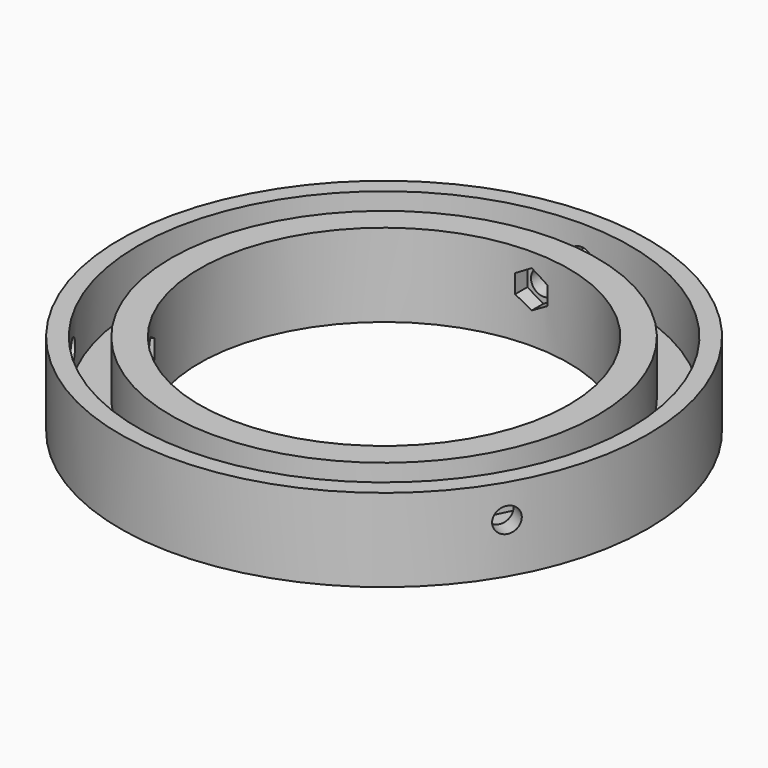
from build123d import *

# Parameters (mm, degrees)
F0_R             = 38.5
F0_R_2           = 33.35
F1_DEPTH         = 15
F2_R             = 44.5
F2_R_2           = 38.5
F3_DEPTH         = 5
F4_R             = 47.7
F4_R_2           = 44.5
F5_DEPTH         = 15
F6_R             = 2.25
F7_DEPTH         = 47.701
F7_COPIES_COUNT  = 3
F10_DEPTH        = 4
F10_COPIES_COUNT = 3


# Not quite as in the source:
# - a pattern or mirror of a feature is missing from the dataset's text; its kind, count and spacing are read off the source's solid


with BuildPart() as f1:
    # F0 (on Top) → F1 (new body)
    with BuildSketch(Plane.XY):
        Circle(F0_R)
        Circle(F0_R_2, mode=Mode.SUBTRACT)
    extrude(amount=F1_DEPTH)

    # F2 (on Top) → F3 (join)
    with BuildSketch(Plane.XY):
        Circle(F2_R)
        Circle(F2_R_2, mode=Mode.SUBTRACT)
    extrude(amount=F3_DEPTH)

    # F4 (on Top) → F5 (join)
    with BuildSketch(Plane.XY):
        Circle(F4_R)
        Circle(F4_R_2, mode=Mode.SUBTRACT)
    extrude(amount=F5_DEPTH)

    # F6 (on Front) → F7 (cut, through all)
    with BuildSketch(Plane.XZ):
        with Locations((0, 9)):
            Circle(F6_R)
    f7 = extrude(amount=-F7_DEPTH, mode=Mode.SUBTRACT)

    # F7_copies: F7 ×3 about axis
    f7_copies_axis = Axis((0, 0, 0), (0, 0, 1))
    for i in range(1, F7_COPIES_COUNT):
        add(f7.rotate(f7_copies_axis, i * 360 / F7_COPIES_COUNT), mode=Mode.SUBTRACT)

    # F9 (on offset) → F10 (cut)
    with BuildSketch(Plane.XZ.offset(-36)):
        Polygon((2.9175, 7.3155805896), (2.9175, 10.6844194104), (0, 12.3688388207), (-2.9175, 10.6844194104), (-2.9175, 7.3155805896), (0, 5.6311611793), align=None)
    f10 = extrude(amount=F10_DEPTH, mode=Mode.SUBTRACT)

    # F10_copies: F10 ×3 about axis
    f10_copies_axis = Axis((0, 0, 0), (0, 0, 1))
    for i in range(1, F10_COPIES_COUNT):
        add(f10.rotate(f10_copies_axis, i * 360 / F10_COPIES_COUNT), mode=Mode.SUBTRACT)


solid = f1.part
